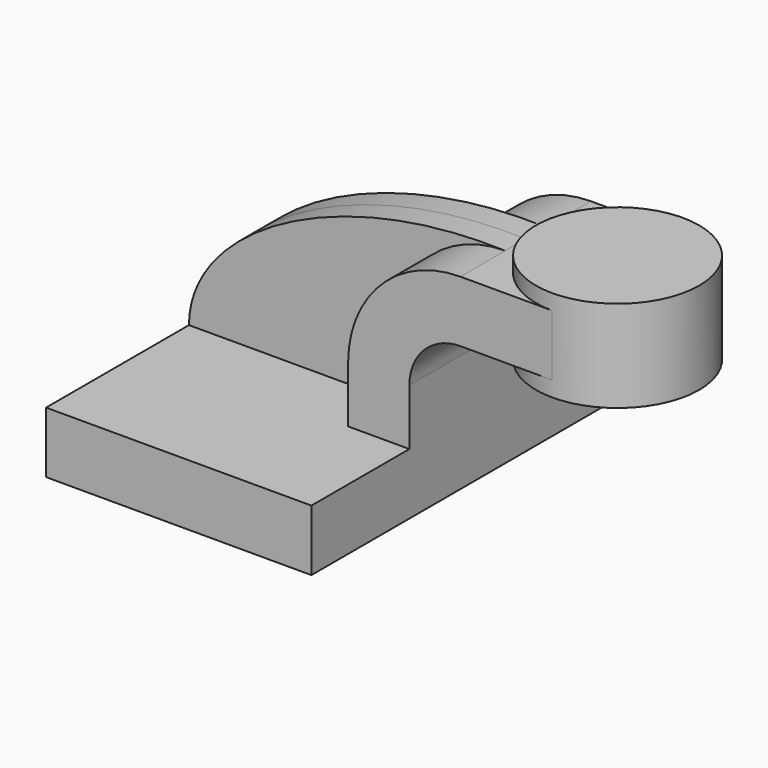
from build123d import *

# Parameters (mm, degrees)
F1_DEPTH = 63.5
F0_W     = 25.4
F0_H     = 19.0246
F2_DEPTH = 25.4
F4_DEPTH = 7.9375


# Not quite as in the source:
# - a feature names something its author has since deleted; it is built from what else it names


with BuildPart() as f1:
    # F0 (on Front) → F1 (new body, symmetric)
    with BuildSketch(Plane.XZ):
        Polygon((-41.275, -9.525), (41.275, -9.525), (41.275, 9.525), (22.225, 9.525), (-41.275, 9.525), align=None)
    extrude(amount=F1_DEPTH, both=True)

    # F0 (on Front) → F2 (join, symmetric)
    with BuildSketch(Plane.XZ):
        with BuildLine():
            Line((22.225, 9.525), (41.275, 9.525))
            Line((41.275, 9.525), (41.275, 27.0002))
            ThreePointArc((41.275, 27.0002), (45.9246798487, 38.2255201513), (57.15, 42.8752))
            Line((57.15, 42.8752), (60.325, 42.8752))
            Line((60.325, 42.8752), (60.325, 61.8998))
            Line((60.325, 61.8998), (57.15, 61.8998))
            ThreePointArc((57.15, 61.8998), (32.4632742898, 51.6794835164), (22.225, 27.0002))
            Line((22.225, 27.0002), (22.225, 9.525))
        make_face()
        with Locations((73.025, 52.3875)):
            Rectangle(F0_W, F0_H)
    extrude(amount=F2_DEPTH, both=True)

    # F0 (on Front) → F3 (revolve)
    with BuildSketch(Plane.XZ):
        Polygon((85.725, 66.675), (85.725, 61.8998), (85.725, 42.8752), (85.725, 38.1), (111.125, 38.1), (111.125, 66.675), align=None)
    revolve(axis=Axis((85.725, 0, 52.3875), (0, 0, -1)))

    # F0 (on Front) → F4 (join, symmetric)
    with BuildSketch(Plane.XZ):
        with BuildLine():
            add(Edge.make_bspline(
                [(-41.275, 9.525), (-41.2365756929, 37.5034026802), (4.0239142254, 63.6744350195), (57.15, 61.8998)],
                knots=[0, 0, 0, 0, 111.4926019969, 111.4926019969, 111.4926019969, 111.4926019969], degree=3))
            Line((-41.275, 9.525), (22.225, 9.525))
            Line((22.225, 9.525), (22.225, 27.0002))
            ThreePointArc((22.225, 27.0002), (32.4632742898, 51.6794835164), (57.15, 61.8998))
        make_face()
    extrude(amount=F4_DEPTH, both=True)


solid = f1.part
